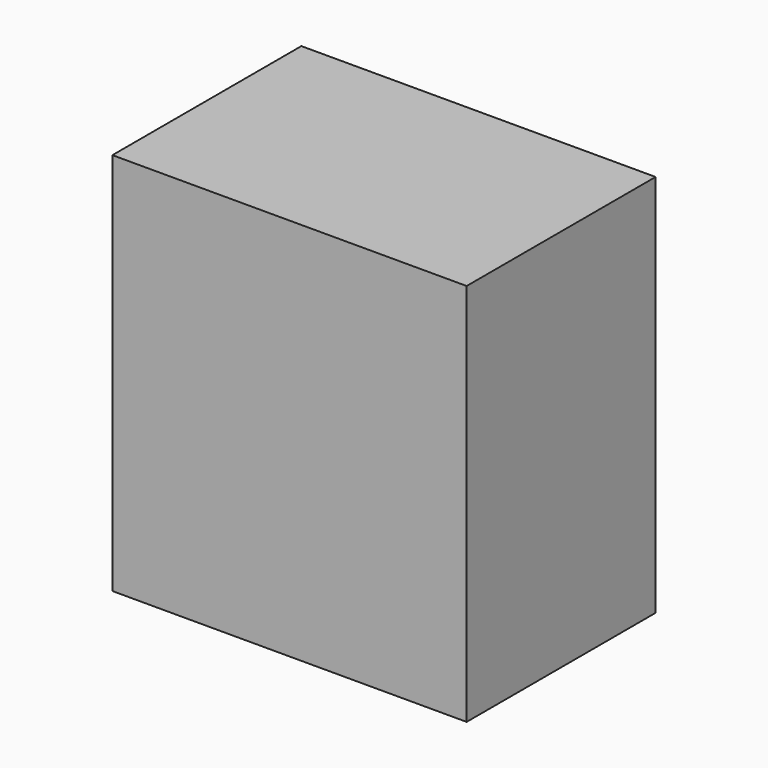
from build123d import *

# Parameters (mm, degrees)
F0_W     = 60
F0_H     = 40
F1_DEPTH = 40
F4_DEPTH = 25


# Not quite as in the source:
# - the program builds the solid bodies; features that only make, move or delete a surface that nothing else refers to are left out


with BuildPart() as f1:
    # F0 (on Top) → F1 (new body)
    with BuildSketch(Plane.XY):
        with Locations((30, -20)):
            Rectangle(F0_W, F0_H)
    extrude(amount=F1_DEPTH)

    # F4 (add): a face of the model
    f4_faces = [f1.faces().sort_by_distance(p)[0] for p in [
        (30, -20, 0),
    ]]
    extrude(f4_faces, amount=F4_DEPTH)


solid = f1.part
